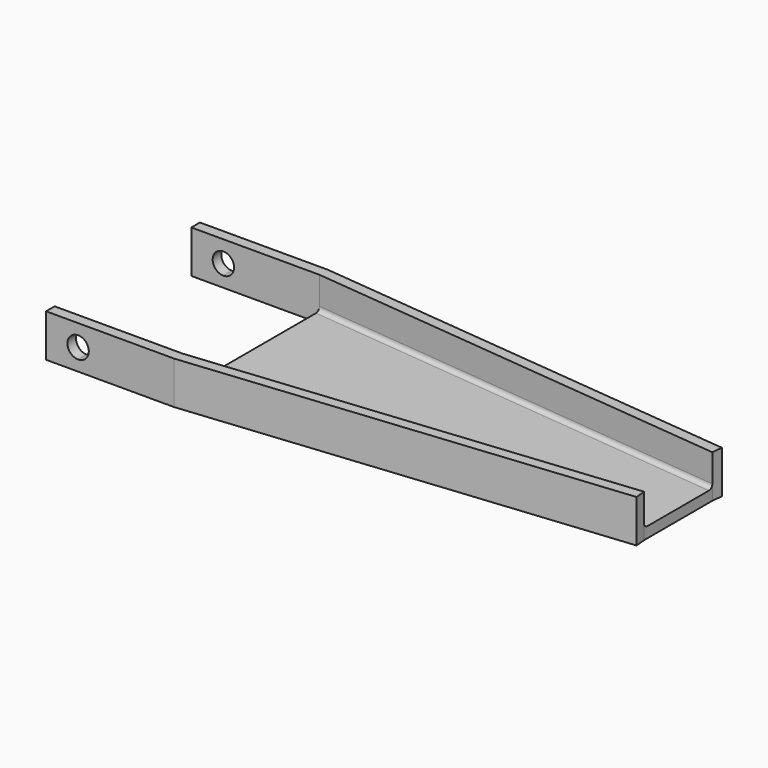
from build123d import *

# Parameters (mm, degrees)
F1_DEPTH = 3.175
F3_DEPTH = 12.7
F5_R     = 1.27
F7_DEPTH = 38.1
F9_DEPTH = 57.1826710194


# Not quite as in the source:
# - a length typed as a fraction of an inch, garbled in the dataset ("3 / 203.2 mm" for 3/8 in), is restored


with BuildPart() as f1:
    # F0 (on Top) → F1 (new body)
    with BuildSketch(Plane.XY):
        Polygon((-63.5, -25.4), (63.5, -12.7), (63.5, 12.7), (-63.5, 25.4), align=None)
    extrude(amount=F1_DEPTH)

    # F2 (on Top) → F3 (join)
    with BuildSketch(Plane.XY):
        Polygon((-63.5, -25.4), (-63.5, -28.5908355097), (63.8159243079, -15.8592430789), (63.5, -12.7), align=None)
    extrude(amount=F3_DEPTH)

    # F4: F1 across plane


with BuildPart() as f1_1:
    add(f1.part)
    add(f1.part.mirror(Plane.XZ))

    # F5
    f5_edges = [f1_1.edges().sort_by_distance(p)[0] for p in [
        (0, -19.05, 3.175),
        (0, 19.05, 3.175),
    ]]
    fillet(f5_edges, radius=F5_R)

    # F6 (on face) → F7 (join)
    with BuildSketch(Plane(origin=(-63.5, 0, 0), x_dir=(0, -1, 0), z_dir=(-1, 0, 0))):
        Polygon((-25.4, 12.7), (-28.5908355097, 12.7), (-28.5908355097, 0), (-25.4, 0), (-25.4, 4.445), align=None)
        Polygon((25.4, 4.445), (25.4, 0), (28.5908355097, 0), (28.5908355097, 12.7), (25.4, 12.7), align=None)
    extrude(amount=F7_DEPTH)

    # F8 (on face) → F9 (cut, through all)
    with BuildSketch(Plane.XZ.offset(28.5908355097)):
        with BuildLine():
            Line((-92.075, 3.175), (-92.075, 9.525))
            ThreePointArc((-92.075, 9.525), (-95.25, 6.35), (-92.075, 3.175))
        make_face()
        with BuildLine():
            ThreePointArc((-88.9, 6.35), (-89.8299359697, 8.5950640303), (-92.075, 9.525))
            Line((-92.075, 9.525), (-92.075, 3.175))
            ThreePointArc((-92.075, 3.175), (-89.8299359697, 4.1049359697), (-88.9, 6.35))
        make_face()
    extrude(amount=-F9_DEPTH, mode=Mode.SUBTRACT)


solid = f1_1.part
